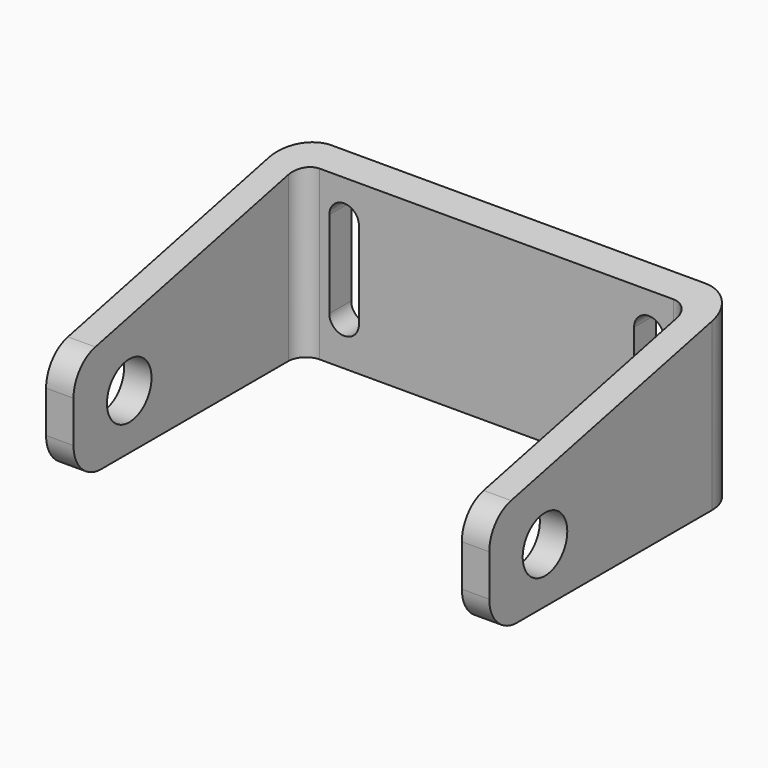
from build123d import *

# Parameters (mm, degrees)
F1_DEPTH      = 12.7
F3_DEPTH      = 16.1615
F3_DEPTH_BACK = 16.1615
F4_R          = 2.032
F5_DEPTH      = 32.322
F5_DEPTH_BACK = 60
F6_R          = 2.54
F8_DEPTH      = 22.861


# Not quite as in the source:
# - an extrude ends at something that could not be found from the text; its depth is read off the source's solid
# - a feature names something its author has since deleted; it is built from what else it names


with BuildPart() as f1:
    # F0 (on Top) → F1 (new body)
    with BuildSketch(Plane.XY):
        with BuildLine():
            Line((13.6205, 0), (0, 0))
            Line((0, 0), (-13.6205, 0))
            ThreePointArc((-13.6205, 0), (-15.4165512242, -0.7439487758), (-16.1605, -2.54))
            Line((-16.1605, -2.54), (-16.1605, -22.86))
            Line((-16.1605, -22.86), (-14.1605, -22.86))
            Line((-14.1605, -22.86), (-14.1605, -3.27))
            ThreePointArc((-14.1605, -3.27), (-13.7885256121, -2.3719743879), (-12.8905, -2))
            Line((-12.8905, -2), (0, -2))
            Line((0, -2), (12.8905, -2))
            ThreePointArc((12.8905, -2), (13.7885256121, -2.3719743879), (14.1605, -3.27))
            Line((14.1605, -3.27), (14.1605, -22.86))
            Line((14.1605, -22.86), (16.1605, -22.86))
            Line((16.1605, -22.86), (16.1605, -2.54))
            ThreePointArc((16.1605, -2.54), (15.4165512242, -0.7439487758), (13.6205, 0))
        make_face()
    extrude(amount=F1_DEPTH)

    # F2 (on Right) → F3 (cut, two sides)
    with BuildSketch(Plane.YZ) as f3_sk:
        Polygon((0, 12.7), (-2.54, 12.7), (-22.86, 12.7), (-22.86, 7.62), align=None)
    extrude(amount=-F3_DEPTH, mode=Mode.SUBTRACT)
    extrude(f3_sk.sketch, amount=F3_DEPTH_BACK, mode=Mode.SUBTRACT)

    # F4 (on face) → F5 (cut, two sides)
    with BuildSketch(Plane.YZ.offset(16.1605)) as f5_sk:
        with Locations((-17.78, 4)):
            Circle(F4_R)
    extrude(amount=-F5_DEPTH, mode=Mode.SUBTRACT)
    extrude(f5_sk.sketch, amount=F5_DEPTH_BACK, mode=Mode.SUBTRACT)

    # F6
    f6_edges = [f1.edges().sort_by_distance(p)[0] for p in [
        (15.1605, -22.86, 7.62),
        (-15.1605, -22.86, 7.62),
        (-15.1605, -22.86, 0),
        (15.1605, -22.86, 0),
    ]]
    fillet(f6_edges, radius=F6_R)

    # F7 (on face) → F8 (cut, through all)
    with BuildSketch(Plane(origin=(0, 0, 0), x_dir=(-1, 0, 0), z_dir=(0, 1, 0))):
        with BuildLine():
            Line((-10.033, 3.175), (-10.033, 9.525))
            ThreePointArc((-10.033, 9.525), (-11.1125, 10.6045), (-12.192, 9.525))
            Line((-12.192, 9.525), (-12.192, 3.175))
            ThreePointArc((-12.192, 3.175), (-11.1125, 2.0955), (-10.033, 3.175))
        make_face()
        with BuildLine():
            ThreePointArc((10.033, 3.175), (11.1125, 2.0955), (12.192, 3.175))
            Line((12.192, 3.175), (12.192, 9.525))
            ThreePointArc((12.192, 9.525), (11.1125, 10.6045), (10.033, 9.525))
            Line((10.033, 9.525), (10.033, 3.175))
        make_face()
    extrude(amount=-F8_DEPTH, mode=Mode.SUBTRACT)


solid = f1.part
